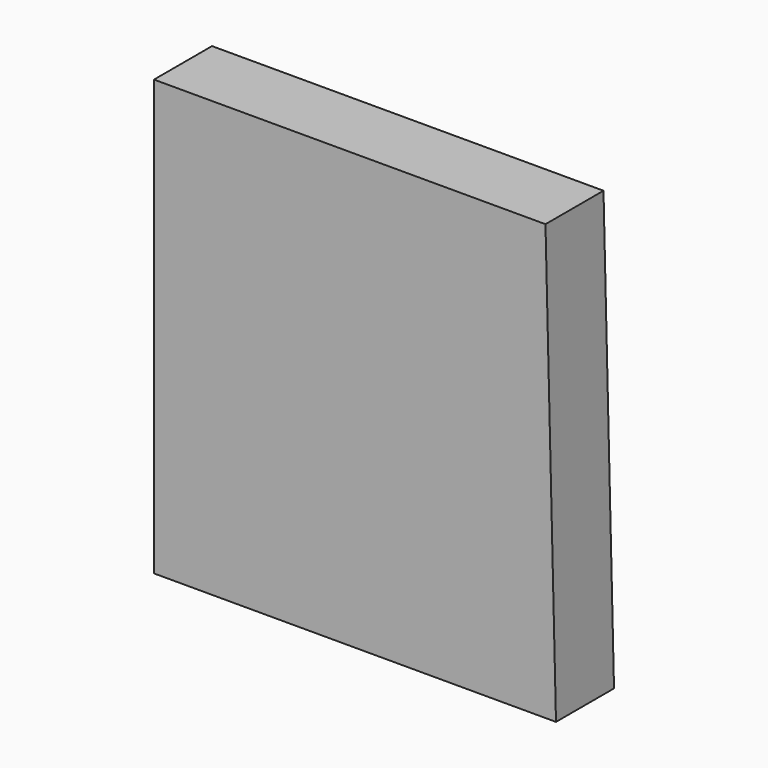
from build123d import *

# Parameters (mm, degrees)
F1_DEPTH = 25.4


# Not quite as in the source:
# - the program builds the solid bodies; features that only make, move or delete a surface that nothing else refers to are left out


with BuildPart() as f1:
    # F0 (on Front) → F1 (new body)
    with BuildSketch(Plane.XZ):
        Polygon((75.7845193148, -77.7228921652), (72.1014291048, 74.5455399156), (-65.0134831667, 74.5455399156), (-65.0134831667, -77.7228921652), align=None)
    extrude(amount=F1_DEPTH)


solid = f1.part
